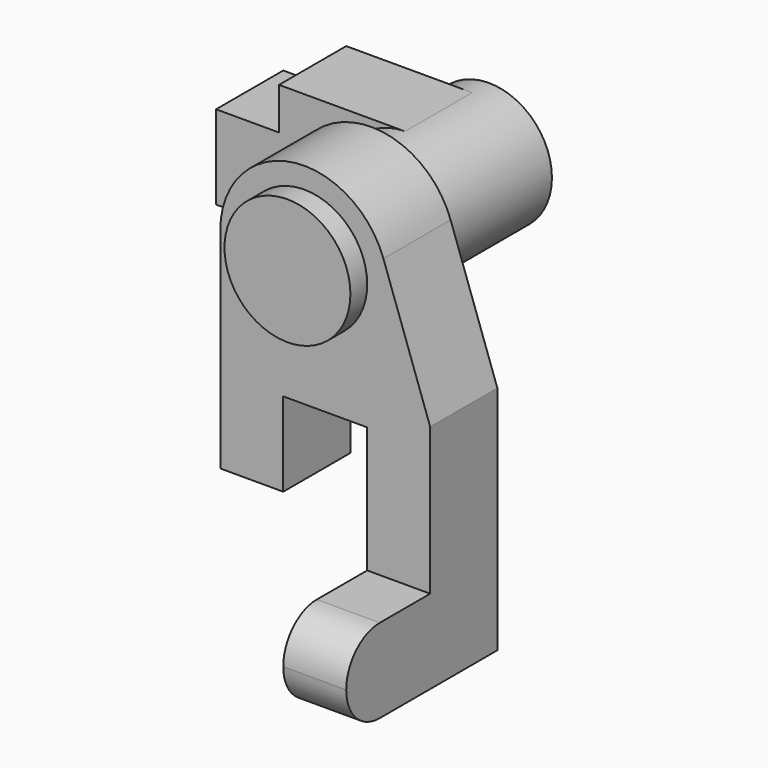
from build123d import *

# Parameters (mm, degrees)
F0_R          = 15
F0_W          = 15
F0_H          = 20
F1_DEPTH      = 20
F2_DEPTH      = 45
F3_DEPTH      = 25
F3_DEPTH_BACK = 35
F4_R          = 9.99999
F6_DEPTH      = 25
F7_DEPTH      = 5


# Not quite as in the source:
# - a fillet or chamfer is up to 0.001 mm smaller than in the source, because OpenCascade refuses the exact size


with BuildPart() as f1:
    # F0 (on Front) → F1 (new body)
    with BuildSketch(Plane.XZ):
        with BuildLine():
            ThreePointArc((-20, 0), (0, -20), (20, 0))
            ThreePointArc((20, 0), (19.7144383856, 3.3676281177), (18.8659080861, 6.6390897033))
            ThreePointArc((18.8659080861, 6.6390897033), (-3.3676281177, 19.7144383856), (-20, 0))
        make_face()
        Circle(F0_R, mode=Mode.SUBTRACT)
        with BuildLine():
            ThreePointArc((18.8659080861, 6.6390897033), (19.7144383856, 3.3676281177), (20, 0))
            ThreePointArc((20, 0), (0, -20), (-20, 0))
            Line((-20, 0), (-20, -50))
            Line((-20, -50), (-5, -50))
            Line((-5, -50), (-5, -30))
            Line((-5, -30), (15, -30))
            Line((15, -30), (15, -60))
            Line((15, -60), (30, -60))
            Line((30, -60), (30, -25))
            Line((30, -25), (18.8659080861, 6.6390897033))
        make_face()
        with Locations((22.5, -70)):
            Rectangle(F0_W, F0_H)
    extrude(amount=F1_DEPTH)

    # F0 (on Front) → F2 (join)
    with BuildSketch(Plane.XZ):
        with Locations((22.5, -70)):
            Rectangle(F0_W, F0_H)
    extrude(amount=F2_DEPTH)

    # F0 (on Front) → F3 (join, two sides)
    with BuildSketch(Plane.XZ) as f3_sk:
        Circle(F0_R)
    extrude(amount=F3_DEPTH)
    extrude(f3_sk.sketch, amount=-F3_DEPTH_BACK)

    # F4 (radius 10 in the source; OpenCascade refuses exactly that, so slightly less here)
    f4_edges = [f1.edges().sort_by_distance(p)[0] for p in [
        (22.5, -45, -60),
        (22.5, -45, -80),
    ]]
    fillet(f4_edges, radius=F4_R)

    # F5 (on face) → F6 (join)
    with BuildSketch(Plane(origin=(0, 35, 0), x_dir=(-1, 0, 0), z_dir=(0, 1, 0))):
        with BuildLine():
            Line((30, 15), (0, 15))
            ThreePointArc((0, 15), (10.6066017178, 10.6066017178), (15, 0))
            ThreePointArc((15, 0), (10.6066017178, -10.6066017178), (0, -15))
            Line((0, -15), (45, -15))
            Line((45, -15), (45, 5))
            Line((45, 5), (30, 5))
            Line((30, 5), (30, 15))
        make_face()
    extrude(amount=-F6_DEPTH)

    # F5 (on face) → F7 (cut)
    with BuildSketch(Plane(origin=(0, 35, 0), x_dir=(-1, 0, 0), z_dir=(0, 1, 0))):
        with BuildLine():
            Line((30, 15), (0, 15))
            ThreePointArc((0, 15), (10.6066017178, 10.6066017178), (15, 0))
            ThreePointArc((15, 0), (10.6066017178, -10.6066017178), (0, -15))
            Line((0, -15), (45, -15))
            Line((45, -15), (45, 5))
            Line((45, 5), (30, 5))
            Line((30, 5), (30, 15))
        make_face()
    extrude(amount=-F7_DEPTH, mode=Mode.SUBTRACT)


solid = f1.part
